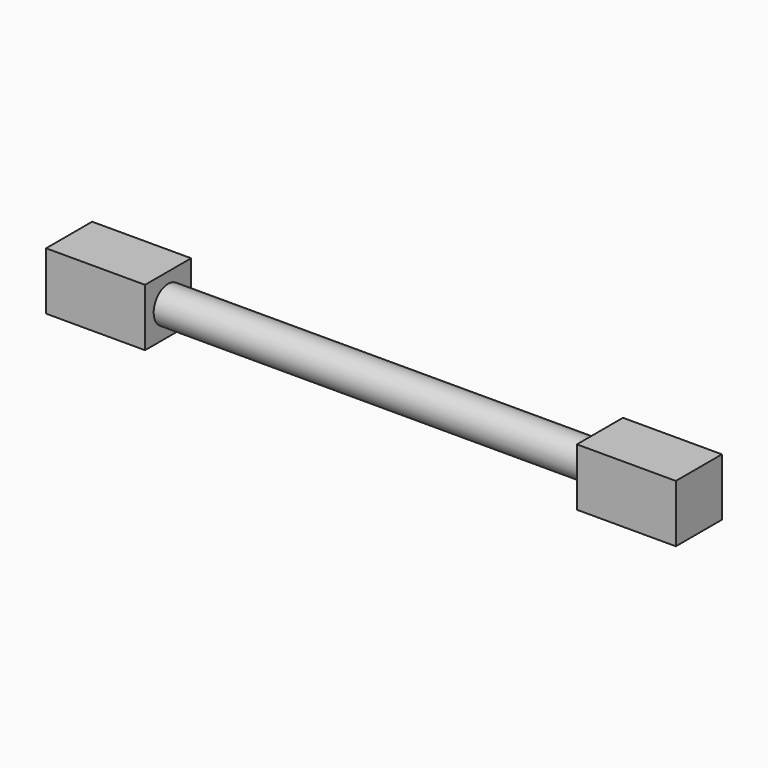
from build123d import *

# Parameters (mm, degrees)
F2_DEPTH = 3.2
F3_DEPTH = 3.2


with BuildPart() as f1:
    # F0 (on Front) → F1 (revolve)
    with BuildSketch(Plane.XZ):
        Polygon((24, 2), (-24, 2), (-24, 0), (0, 0), (24, 0), align=None)
    revolve(axis=Axis((-12, 0, 0), (1, 0, 0)))


with BuildPart() as f2:
    # F0 (on Front) → F2 (new body, symmetric)
    with BuildSketch(Plane.XZ):
        Polygon((-24, 3.2), (-35, 3.2), (-35, -3.2), (-24, -3.2), (-24, 0), (-24, 2), align=None)
    extrude(amount=F2_DEPTH, both=True)


with BuildPart() as f3:
    # F0 (on Front) → F3 (new body, symmetric)
    with BuildSketch(Plane.XZ):
        Polygon((35, 3.2), (24, 3.2), (24, 2), (24, 0), (24, -3.2), (35, -3.2), align=None)
    extrude(amount=F3_DEPTH, both=True)


solid = Compound([f1.part, f2.part, f3.part])
